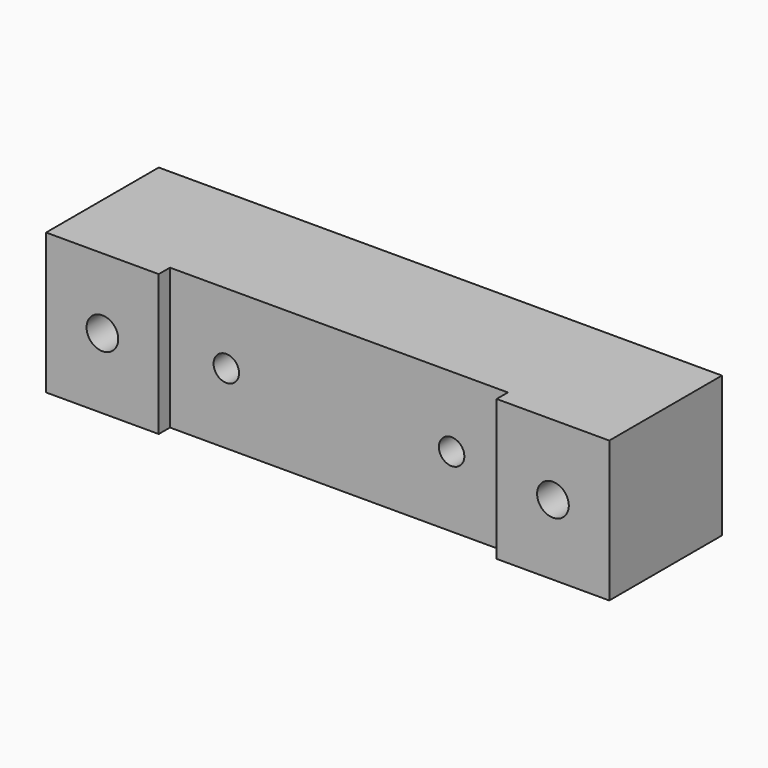
from build123d import *

# Parameters (mm, degrees)
F0_W     = 63.5
F0_H     = 63.5
F1_DEPTH = 127
F3_D     = 14.2875
F4_W     = 152.4
F4_H     = 63.5
F5_DEPTH = 6.35
F7_D     = 11.50874
F7_DEPTH = 38.1
F7_TIP   = 3.4575743203


# Not quite as in the source:
# - a length typed as a fraction of an inch, garbled in the dataset ("3 / 203.2 mm" for 3/8 in), is restored


with BuildPart() as f1:
    # F0 (on Right) → F1 (new body, symmetric)
    with BuildSketch(Plane.YZ):
        Rectangle(F0_W, F0_H)
    extrude(amount=F1_DEPTH, both=True)

    # F3 (through all)
    with Locations(Plane.XZ.offset(31.75)):
        with Locations((-101.6, 0), (101.6, 0)):
            Hole(F3_D / 2)

    # F4 (on face) → F5 (cut)
    with BuildSketch(Plane.XZ.offset(31.75)):
        Rectangle(F4_W, F4_H)
    extrude(amount=-F5_DEPTH, mode=Mode.SUBTRACT)

    # F7
    with Locations(Plane.XZ.offset(25.4)):
        with Locations((-50.8, 0), (50.8, 0)):
            Hole(F7_D / 2, depth=F7_DEPTH)
            with Locations((0, 0, -(F7_DEPTH + F7_TIP / 2))):  # 118° drill point
                Cone(0, F7_D / 2, F7_TIP, mode=Mode.SUBTRACT)


solid = f1.part
